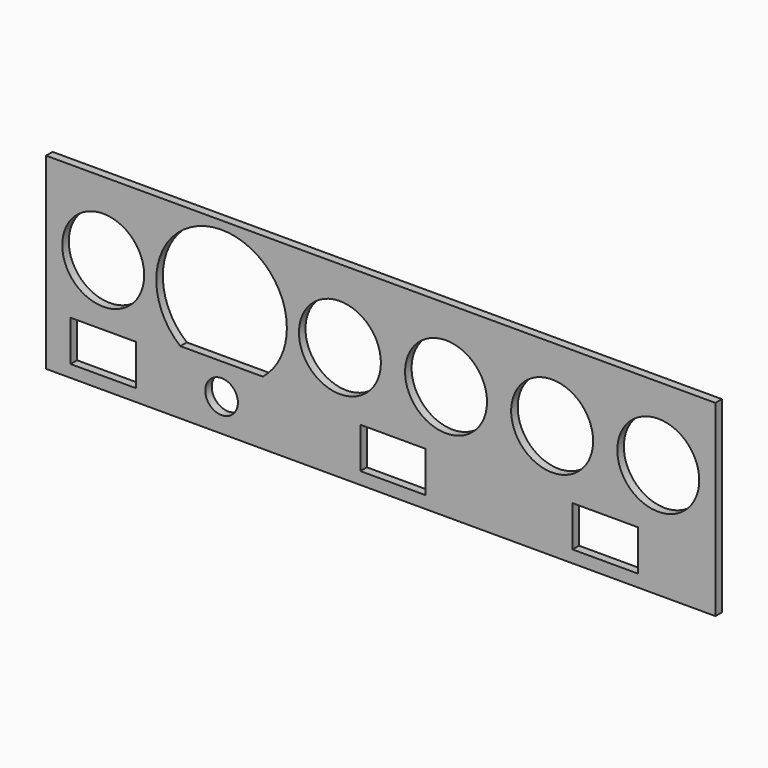
from build123d import *

# Parameters (mm, degrees)
F0_W      = 520.7
F0_H      = 146.05
F0_R      = 31.877
F1_DEPTH  = 6.35
F2_DEPTH  = 6.35
F3_R      = 10.0959291711
F3_R_2    = 9.3516208714
F3_R_3    = 9.399866871
F4_DEPTH  = 25.4
F5_R      = 2.413
F6_DEPTH  = 25.4
F7_W      = 6.35
F7_H      = 6.35
F8_DEPTH  = 25.4
F9_W      = 50.8
F9_H      = 31.75
F10_DEPTH = 25.4
F11_R     = 12.7
F12_DEPTH = 12.7


# Not quite as in the source:
# - a feature names something its author has since deleted; it is built from what else it names


with BuildPart() as f1:
    # F0 (on Front) → F1 (new body)
    with BuildSketch(Plane.XZ):
        with Locations((0.0123051805, 73.0250019237)):
            Rectangle(F0_W, F0_H)
        with Locations((-215.8876948195, 88.9000019237)):
            Circle(F0_R, mode=Mode.SUBTRACT)
        with BuildLine():
            ThreePointArc((-155.9332892075, 49.5438408284), (-145.5947264636, 134.7931724118), (-73.0126948195, 88.9000019237))
            ThreePointArc((-73.0126948195, 88.9000019237), (-77.9195243313, 67.1179702796), (-91.6921004315, 49.5438408284))
            ThreePointArc((-91.6921004315, 49.5438408284), (-123.8126948195, 38.1000019237), (-155.9332892075, 49.5438408284))
        make_face(mode=Mode.SUBTRACT)
        with Locations((-31.7376948195, 88.9000019237)):
            Circle(F0_R, mode=Mode.SUBTRACT)
        with Locations((50.8123051805, 88.9000019237)):
            Circle(F0_R, mode=Mode.SUBTRACT)
        with Locations((133.3623051805, 88.9000019237)):
            Circle(F0_R, mode=Mode.SUBTRACT)
        with Locations((215.9123051805, 88.9000019237)):
            Circle(F0_R, mode=Mode.SUBTRACT)
    extrude(amount=F1_DEPTH)

    # F0 (on Front) → F2 (join)
    with BuildSketch(Plane.XZ):
        with BuildLine():
            Line((-91.6921004315, 49.5438408284), (-155.9332892075, 49.5438408284))
            ThreePointArc((-155.9332892075, 49.5438408284), (-123.8126948195, 38.1000019237), (-91.6921004315, 49.5438408284))
        make_face()
    extrude(amount=F2_DEPTH)

    # F3 (on face) → F4 (cut)
    with BuildSketch(Plane.XZ.offset(6.35)):
        with Locations((-215.8876948195, 25.4000019237)):
            Circle(F3_R)
        with Locations((9.5373051805, 25.4000019237)):
            Circle(F3_R_2)
        with Locations((174.6373051805, 25.4000019237)):
            Circle(F3_R_3)
    extrude(amount=-F4_DEPTH, mode=Mode.SUBTRACT)

    # F5 (on face) → F6 (cut)
    with BuildSketch(Plane.XZ.offset(6.35)):
        with Locations((-155.5626948195, 120.6500019237)):
            Circle(F5_R)
        with Locations((-92.0626948195, 120.6500019237)):
            Circle(F5_R)
        with Locations((-92.0626948195, 57.1500019237)):
            Circle(F5_R)
        with Locations((-155.5626948195, 57.1500019237)):
            Circle(F5_R)
    extrude(amount=-F6_DEPTH, mode=Mode.SUBTRACT)

    # F7 (on face) → F8 (cut)
    with BuildSketch(Plane.XZ.offset(6.35)):
        with Locations((-269.875, 142.875)):
            Rectangle(F7_W, F7_H)
        with Locations((269.875, 142.875)):
            Rectangle(F7_W, F7_H)
    extrude(amount=-F8_DEPTH, mode=Mode.SUBTRACT)

    # F9 (on face) → F10 (cut)
    with BuildSketch(Plane.XZ.offset(6.35)):
        with Locations((-215.8876948195, 25.4000019237)):
            Rectangle(F9_W, F9_H)
        with Locations((9.5373051805, 25.4000019237)):
            Rectangle(F9_W, F9_H)
        with Locations((174.6373051805, 25.4000019237)):
            Rectangle(F9_W, F9_H)
    extrude(amount=-F10_DEPTH, mode=Mode.SUBTRACT)

    # F11 (on face) → F12 (cut, symmetric)
    with BuildSketch(Plane.XZ.offset(6.35)):
        with Locations((-123.8126948195, 25.4000019237)):
            Circle(F11_R)
    extrude(amount=F12_DEPTH, both=True, mode=Mode.SUBTRACT)


solid = f1.part
